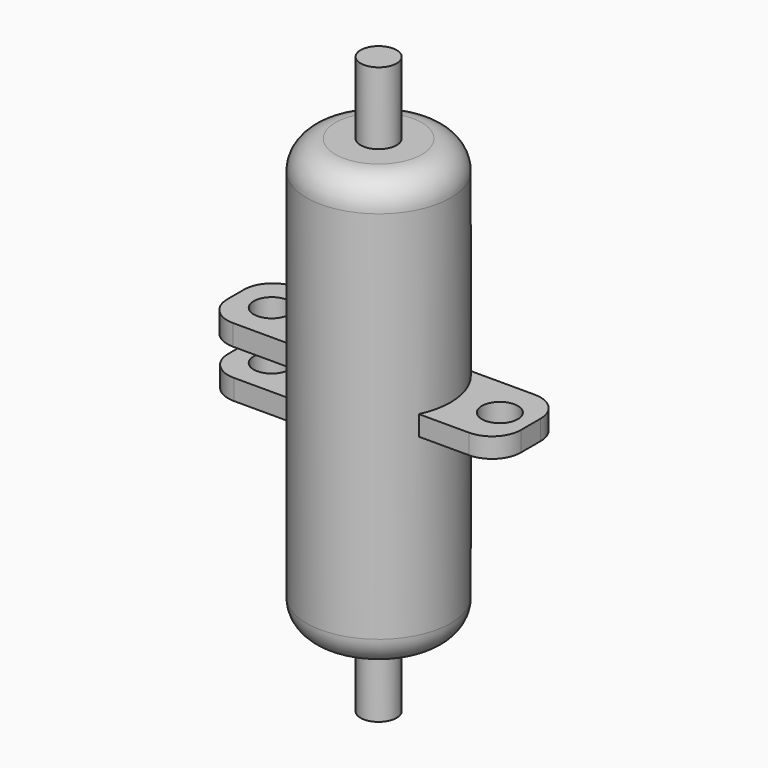
from build123d import *

# Parameters (mm, degrees)
F0_R      = 50
F1_DEPTH  = 300
F2_W      = 54.253433831
F2_H      = 14.4457370043
F2_W_2    = 52.9929734766
F2_H_2    = 14.163993299
F3_DEPTH  = 100
F4_W      = 57.0899797603
F4_H      = 13.7881338596
F5_DEPTH  = 100
F6_R      = 12.5
F7_DEPTH  = 158.7383495102
F8_R      = 12.5
F9_DEPTH  = 176.0267437825
F10_R     = 20
F11_R     = 20
F12_R     = 12.5
F13_DEPTH = 50
F14_R     = 12.5
F15_DEPTH = 50


with BuildPart() as f1:
    # F0 (on Top) → F1 (new body)
    with BuildSketch(Plane.XY):
        Circle(F0_R)
    extrude(amount=F1_DEPTH)

    # F2 (on Right) → F3 (join)
    with BuildSketch(Plane.YZ):
        with Locations((0.9253951721, 164.6268591285)):
            Rectangle(F2_W, F2_H)
        with Locations((0.9205453098, 131.056252867)):
            Rectangle(F2_W_2, F2_H_2)
    extrude(amount=-F3_DEPTH)

    # F4 (on Right) → F5 (join)
    with BuildSketch(Plane.YZ):
        with Locations((6.9804289378, 148.1567174196)):
            Rectangle(F4_W, F4_H)
    extrude(amount=F5_DEPTH)

    # F6 (on face) → F7 (cut, through all)
    with BuildSketch(Plane(origin=(0, 0, 141.2626504898), x_dir=(1, 0, 0), z_dir=(0, 0, -1))):
        with Locations((78.2878473401, -7.3254397139)):
            Circle(F6_R)
    extrude(amount=-F7_DEPTH, mode=Mode.SUBTRACT)

    # F8 (on face) → F9 (cut, through all)
    with BuildSketch(Plane(origin=(0, 0, 123.9742562175), x_dir=(1, 0, 0), z_dir=(0, 0, -1))):
        with Locations((-74.919745326, -0.9205453098)):
            Circle(F8_R)
    extrude(amount=-F9_DEPTH, mode=Mode.SUBTRACT)

    # F10
    f10_edges = [f1.edges().sort_by_distance(p)[0] for p in [
        (-50, 0, 300),
        (-50, 0, 0),
    ]]
    fillet(f10_edges, radius=F10_R)

    # F11
    f11_edges = [f1.edges().sort_by_distance(p)[0] for p in [
        (100, 35.525419, 148.156717),
        (100, -21.564561, 148.156717),
        (-100, -25.575941, 131.056253),
        (-100, 27.417032, 131.056253),
        (-100, -26.201322, 164.626859),
        (-100, 28.052112, 164.626859),
    ]]
    fillet(f11_edges, radius=F11_R)

    # F12 (on face) → F13 (join)
    with BuildSketch(Plane.XY.offset(300)):
        Circle(F12_R)
    extrude(amount=F13_DEPTH)

    # F14 (on face) → F15 (join)
    with BuildSketch(Plane(origin=(0, 0, 0), x_dir=(1, 0, 0), z_dir=(0, 0, -1))):
        Circle(F14_R)
    extrude(amount=F15_DEPTH)


solid = f1.part
